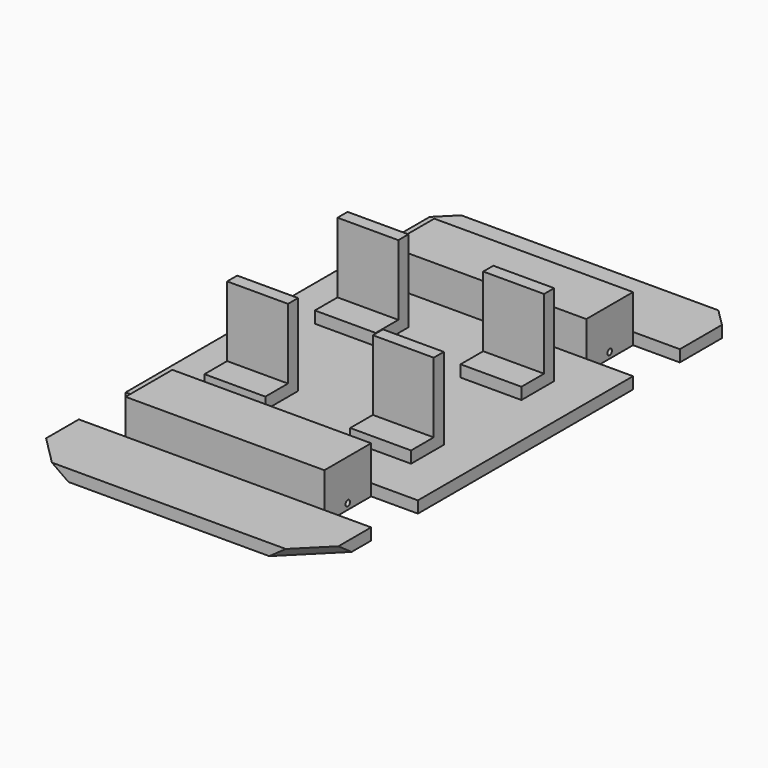
from build123d import *

# Parameters (mm, degrees)
F1_DEPTH  = 1
F2_W      = 5
F2_H      = 3
F3_DEPTH  = 8.5
F4_SIZE   = 2.5
F5_SIZE   = 1.5
F6_SIZE   = 0.99999
F7_R      = 0.245
F8_DEPTH  = 17
F9_W      = 5.2027019071
F9_H      = 3.5
F10_DEPTH = 1
F11_W     = 5.2027019071
F11_H     = 1.0782994613
F12_DEPTH = 6
F13_W     = 5.2027019071
F13_H     = 1.0795953252
F14_DEPTH = 6


# Not quite as in the source:
# - a fillet or chamfer is up to 0.001 mm smaller than in the source, because OpenCascade refuses the exact size


with BuildPart() as f1:
    # F0 (on Top) → F1 (new body)
    with BuildSketch(Plane.XY):
        Polygon((-12.5, -22.5), (12.5, -22.5), (12.5, -16.5), (8.5, -16.5), (8.5, -11.5), (12.5, -11.5), (12.5, 11.5), (8.5, 11.5), (8.5, 16.5), (12.5, 16.5), (12.5, 22.5), (-12.5, 22.5), (-12.5, 16.5), (-8.5, 16.5), (-8.5, 11.5), (-12.5, 11.5), (-12.5, -11.5), (-8.5, -11.5), (-8.5, -16.5), (-12.5, -16.5), align=None)
    extrude(amount=F1_DEPTH)

    # F2 (on Right) → F3 (join, symmetric)
    with BuildSketch(Plane.YZ):
        with Locations((-14, 2.5)):
            Rectangle(F2_W, F2_H)
        with Locations((14, 2.5)):
            Rectangle(F2_W, F2_H)
    extrude(amount=F3_DEPTH, both=True)

    # F4
    f4_edges = [f1.edges().sort_by_distance(p)[0] for p in [
        (12.5, -22.5, 0.5),
        (-12.5, -22.5, 0.5),
    ]]
    chamfer(f4_edges, length=F4_SIZE)

    # F5
    f5_edges = [f1.edges().sort_by_distance(p)[0] for p in [
        (12.5, 22.5, 0.5),
        (-12.5, 22.5, 0.5),
    ]]
    chamfer(f5_edges, length=F5_SIZE)

    # F6 (size 1 in the source; OpenCascade refuses exactly that, so slightly less here)
    f6_edges = [f1.edges().sort_by_distance(p)[0] for p in [
        (-11.25, -21.25, 0),
        (11.25, -21.25, 0),
    ]]
    chamfer(f6_edges, length=F6_SIZE)

    # F7 (on face) → F8 (cut)
    with BuildSketch(Plane.YZ.offset(8.5)):
        with Locations((-14, 0.5039868411)):
            Circle(F7_R)
        with Locations((14, 0.5039868411)):
            Circle(F7_R)
    extrude(amount=-F8_DEPTH, mode=Mode.SUBTRACT)

    # F9 (on face) → F10 (join)
    with BuildSketch(Plane.XY.offset(1)):
        with Locations((6.2317421885, -5.8993692152)):
            Rectangle(F9_W, F9_H)
        with Locations((-6.2317421885, -5.8993692152)):
            Rectangle(F9_W, F9_H)
        with Locations((-6.2317421885, 5.8993692152)):
            Rectangle(F9_W, F9_H)
        with Locations((6.2317421885, 5.8993692152)):
            Rectangle(F9_W, F9_H)
    extrude(amount=F10_DEPTH)

    # F11 (on face) → F12 (join)
    with BuildSketch(Plane.XY.offset(2)):
        with Locations((6.2317421885, -4.6885189459)):
            Rectangle(F11_W, F11_H)
        with Locations((-6.2317421885, -4.6885189459)):
            Rectangle(F11_W, F11_H)
    extrude(amount=F12_DEPTH)

    # F13 (on face) → F14 (join)
    with BuildSketch(Plane.XY.offset(2)):
        with Locations((6.2317421885, 7.1095715527)):
            Rectangle(F13_W, F13_H)
        with Locations((-6.2317421885, 7.1095715527)):
            Rectangle(F13_W, F13_H)
    extrude(amount=F14_DEPTH)


solid = f1.part
